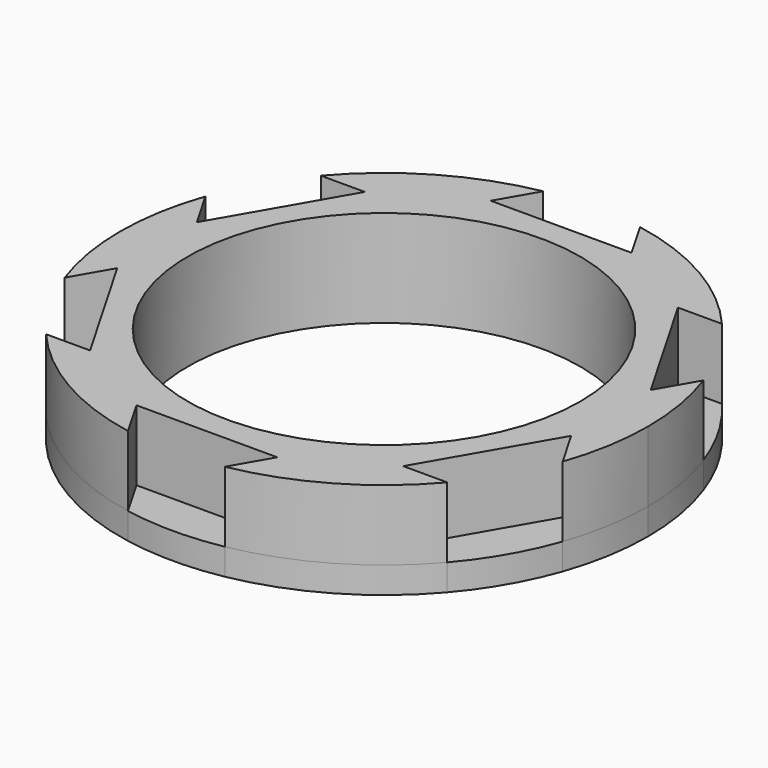
from build123d import *

# Parameters (mm, degrees)
F0_R     = 11.15
F1_DEPTH = 4
F3_DEPTH = 16.2
F4_R     = 11.15
F5_DEPTH = 1.5


with BuildPart() as f1:
    # F0 (on Top) → F1 (new body)
    with BuildSketch(Plane.XY):
        with BuildLine():
            ThreePointArc((-2.75, 14.7457621031), (-9.5851447563, -11.5379807592), (15, 0))
            ThreePointArc((15, 0), (11.5379807592, 9.5851447563), (2.75, 14.7457621031))
            Line((2.75, 14.7457621031), (4, 12.5806985936))
            Line((4, 12.5806985936), (0, 12.5806985936))
            Line((0, 12.5806985936), (-4, 12.5806985936))
            Line((-4, 12.5806985936), (-2.75, 14.7457621031))
        make_face()
        Circle(F0_R, mode=Mode.SUBTRACT)
        with BuildLine():
            Line((4, 12.5806985936), (2.75, 14.7457621031))
            ThreePointArc((2.75, 14.7457621031), (0, 15), (-2.75, 14.7457621031))
            Line((-2.75, 14.7457621031), (-4, 12.5806985936))
            Line((-4, 12.5806985936), (0, 12.5806985936))
            Line((0, 12.5806985936), (4, 12.5806985936))
        make_face()
    extrude(amount=F1_DEPTH)

    # F2 (on face) → F3 (cut)
    with BuildSketch(Plane.XY.offset(4)):
        with BuildLine():
            ThreePointArc((-11.3952045794, 9.7544509119), (-12.9903810568, 7.5), (-14.1452045794, 4.9913111911))
            Line((-14.1452045794, 4.9913111911), (-12.8952045794, 2.8262476817))
            Line((-12.8952045794, 2.8262476817), (-8.8952045794, 9.7544509119))
            Line((-8.8952045794, 9.7544509119), (-11.3952045794, 9.7544509119))
        make_face()
        with BuildLine():
            Line((-12.8952045794, -2.8262476817), (-14.1452045794, -4.9913111911))
            ThreePointArc((-14.1452045794, -4.9913111911), (-12.9903810568, -7.5), (-11.3952045794, -9.7544509119))
            Line((-11.3952045794, -9.7544509119), (-8.8952045794, -9.7544509119))
            Line((-8.8952045794, -9.7544509119), (-12.8952045794, -2.8262476817))
        make_face()
        with BuildLine():
            Line((-4, -12.5806985936), (-2.75, -14.7457621031))
            ThreePointArc((-2.75, -14.7457621031), (0, -15), (2.75, -14.7457621031))
            Line((2.75, -14.7457621031), (4, -12.5806985936))
            Line((4, -12.5806985936), (-4, -12.5806985936))
        make_face()
        with BuildLine():
            Line((8.8952045794, -9.7544509119), (11.3952045794, -9.7544509119))
            ThreePointArc((11.3952045794, -9.7544509119), (12.9903810568, -7.5), (14.1452045794, -4.9913111911))
            Line((14.1452045794, -4.9913111911), (12.8952045794, -2.8262476817))
            Line((12.8952045794, -2.8262476817), (8.8952045794, -9.7544509119))
        make_face()
        with BuildLine():
            ThreePointArc((14.1452045794, 4.9913111911), (12.9903810568, 7.5), (11.3952045794, 9.7544509119))
            Line((11.3952045794, 9.7544509119), (8.8952045794, 9.7544509119))
            Line((8.8952045794, 9.7544509119), (12.8952045794, 2.8262476817))
            Line((12.8952045794, 2.8262476817), (14.1452045794, 4.9913111911))
        make_face()
        with BuildLine():
            ThreePointArc((2.75, 14.7457621031), (0, 15), (-2.75, 14.7457621031))
            Line((-2.75, 14.7457621031), (-4, 12.5806985936))
            Line((-4, 12.5806985936), (4, 12.5806985936))
            Line((4, 12.5806985936), (2.75, 14.7457621031))
        make_face()
    extrude(amount=-F3_DEPTH, mode=Mode.SUBTRACT)

    # F4 (on face) → F5 (join)
    with BuildSketch(Plane(origin=(0, 0, 0), x_dir=(1, 0, 0), z_dir=(0, 0, -1))):
        with BuildLine():
            ThreePointArc((14.1452045794, -4.9913111911), (14.784756824, -2.5319884783), (15, 0))
            ThreePointArc((15, 0), (14.784756824, 2.5319884783), (14.1452045794, 4.9913111911))
            Line((14.1452045794, 4.9913111911), (12.8952045794, 2.8262476817))
            Line((12.8952045794, 2.8262476817), (8.8952045794, 9.7544509119))
            Line((8.8952045794, 9.7544509119), (11.3952045794, 9.7544509119))
            ThreePointArc((11.3952045794, 9.7544509119), (7.5, 12.9903810568), (2.75, 14.7457621031))
            Line((2.75, 14.7457621031), (4, 12.5806985936))
            Line((4, 12.5806985936), (-4, 12.5806985936))
            Line((-4, 12.5806985936), (-2.75, 14.7457621031))
            ThreePointArc((-2.75, 14.7457621031), (-7.5, 12.9903810568), (-11.3952045794, 9.7544509119))
            Line((-11.3952045794, 9.7544509119), (-8.8952045794, 9.7544509119))
            Line((-8.8952045794, 9.7544509119), (-12.8952045794, 2.8262476817))
            Line((-12.8952045794, 2.8262476817), (-14.1452045794, 4.9913111911))
            ThreePointArc((-14.1452045794, 4.9913111911), (-15, 0), (-14.1452045794, -4.9913111911))
            Line((-14.1452045794, -4.9913111911), (-12.8952045794, -2.8262476817))
            Line((-12.8952045794, -2.8262476817), (-8.8952045794, -9.7544509119))
            Line((-8.8952045794, -9.7544509119), (-11.3952045794, -9.7544509119))
            ThreePointArc((-11.3952045794, -9.7544509119), (-7.5, -12.9903810568), (-2.75, -14.7457621031))
            Line((-2.75, -14.7457621031), (-4, -12.5806985936))
            Line((-4, -12.5806985936), (4, -12.5806985936))
            Line((4, -12.5806985936), (2.75, -14.7457621031))
            ThreePointArc((2.75, -14.7457621031), (7.5, -12.9903810568), (11.3952045794, -9.7544509119))
            Line((11.3952045794, -9.7544509119), (8.8952045794, -9.7544509119))
            Line((8.8952045794, -9.7544509119), (12.8952045794, -2.8262476817))
            Line((12.8952045794, -2.8262476817), (14.1452045794, -4.9913111911))
        make_face()
        Circle(F4_R, mode=Mode.SUBTRACT)
        with BuildLine():
            Line((12.8952045794, 2.8262476817), (14.1452045794, 4.9913111911))
            ThreePointArc((14.1452045794, 4.9913111911), (12.9903810568, 7.5), (11.3952045794, 9.7544509119))
            Line((11.3952045794, 9.7544509119), (8.8952045794, 9.7544509119))
            Line((8.8952045794, 9.7544509119), (12.8952045794, 2.8262476817))
        make_face()
        with BuildLine():
            ThreePointArc((11.3952045794, -9.7544509119), (12.9903810568, -7.5), (14.1452045794, -4.9913111911))
            Line((14.1452045794, -4.9913111911), (12.8952045794, -2.8262476817))
            Line((12.8952045794, -2.8262476817), (8.8952045794, -9.7544509119))
            Line((8.8952045794, -9.7544509119), (11.3952045794, -9.7544509119))
        make_face()
        with BuildLine():
            Line((4, 12.5806985936), (2.75, 14.7457621031))
            ThreePointArc((2.75, 14.7457621031), (0, 15), (-2.75, 14.7457621031))
            Line((-2.75, 14.7457621031), (-4, 12.5806985936))
            Line((-4, 12.5806985936), (4, 12.5806985936))
        make_face()
        with BuildLine():
            ThreePointArc((-2.75, -14.7457621031), (0, -15), (2.75, -14.7457621031))
            Line((2.75, -14.7457621031), (4, -12.5806985936))
            Line((4, -12.5806985936), (-4, -12.5806985936))
            Line((-4, -12.5806985936), (-2.75, -14.7457621031))
        make_face()
        with BuildLine():
            Line((-8.8952045794, 9.7544509119), (-11.3952045794, 9.7544509119))
            ThreePointArc((-11.3952045794, 9.7544509119), (-12.9903810568, 7.5), (-14.1452045794, 4.9913111911))
            Line((-14.1452045794, 4.9913111911), (-12.8952045794, 2.8262476817))
            Line((-12.8952045794, 2.8262476817), (-8.8952045794, 9.7544509119))
        make_face()
        with BuildLine():
            ThreePointArc((-14.1452045794, -4.9913111911), (-12.9903810568, -7.5), (-11.3952045794, -9.7544509119))
            Line((-11.3952045794, -9.7544509119), (-8.8952045794, -9.7544509119))
            Line((-8.8952045794, -9.7544509119), (-12.8952045794, -2.8262476817))
            Line((-12.8952045794, -2.8262476817), (-14.1452045794, -4.9913111911))
        make_face()
    extrude(amount=F5_DEPTH)


solid = f1.part
